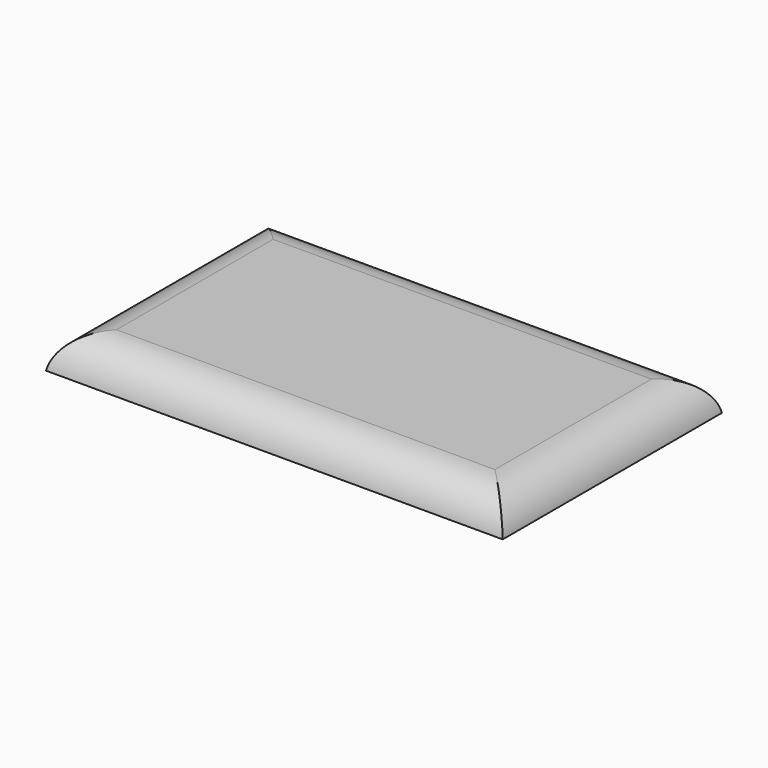
from build123d import *

# Parameters (mm, degrees)
F0_W        = 63.5
F0_H        = 38.1
F1_DEPTH    = 4.572
F2_T1_DEPTH = 65.285274649
F2_T3_DEPTH = 90.685274649


# Not quite as in the source:
# - a fillet or chamfer that OpenCascade refuses, or shapes differently, is made with other operations: its cross-section is extruded or revolved along the edge and cut away or added
# - the program builds the solid bodies; features that only make, move or delete a surface that nothing else refers to are left out


with BuildPart() as f1:
    # F0 (on Top) → F1 (new body)
    with BuildSketch(Plane.XY):
        Rectangle(F0_W, F0_H)
    extrude(amount=F1_DEPTH)

    # F2: fillet of radius 5.5188922036 on 4 edges, made by hand

    # F2_s2 → F2_t1 (cut)
    with BuildSketch(Plane.XZ.offset(-32.6426373245)):
        with BuildLine():
            ThreePointArc((-31.75, 0), (-29.8648723748, 3.2770850191), (-26.3129450702, 4.572))
            Line((-26.3129450702, 4.572), (-31.75, 4.572))
            Line((-31.75, 4.572), (-31.75, 0))
        make_face()
        with BuildLine():
            ThreePointArc((31.75, 0), (29.8648723748, 3.2770850191), (26.3129450702, 4.572))
            Line((26.3129450702, 4.572), (31.75, 4.572))
            Line((31.75, 4.572), (31.75, 0))
        make_face()
    extrude(amount=F2_T1_DEPTH, mode=Mode.SUBTRACT)

    # F2_s4 → F2_t3 (cut)
    with BuildSketch(Plane.YZ.offset(-45.3426373245)):
        with BuildLine():
            ThreePointArc((-19.05, 0), (-17.1648723748, 3.2770850191), (-13.6129450702, 4.572))
            Line((-13.6129450702, 4.572), (-19.05, 4.572))
            Line((-19.05, 4.572), (-19.05, 0))
        make_face()
        with BuildLine():
            ThreePointArc((19.05, 0), (17.1648723748, 3.2770850191), (13.6129450702, 4.572))
            Line((13.6129450702, 4.572), (19.05, 4.572))
            Line((19.05, 4.572), (19.05, 0))
        make_face()
    extrude(amount=F2_T3_DEPTH, mode=Mode.SUBTRACT)


solid = f1.part
